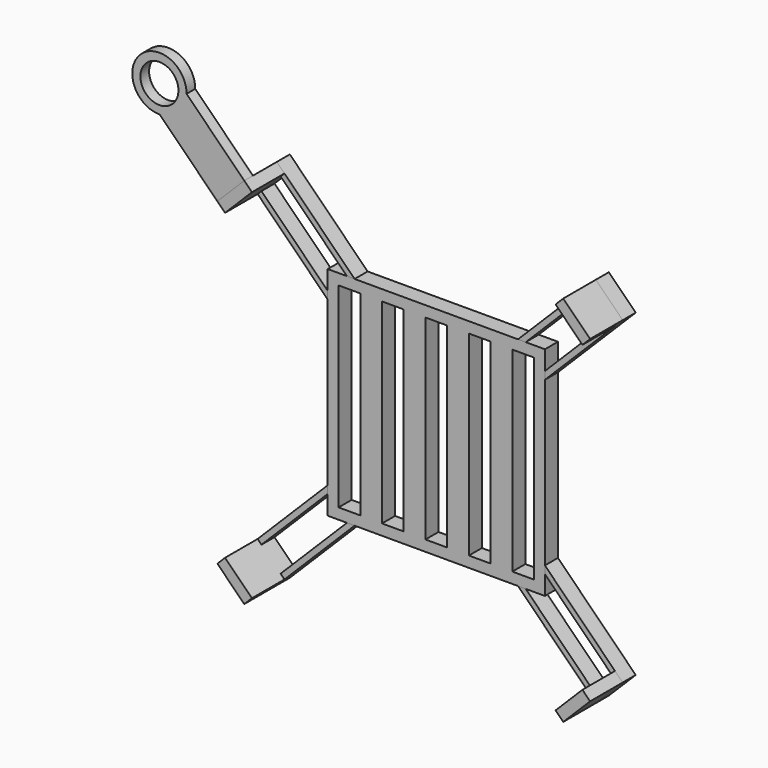
from build123d import *

# Parameters (mm, degrees)
F0_W      = 40
F0_H      = 40
F0_W_2    = 4
F0_H_2    = 36
F1_DEPTH  = 3
F3_DEPTH  = 3
F4_DEPTH  = 25
F5_DEPTH  = 25
F6_DEPTH  = 25
F7_DEPTH  = 25
F9_DEPTH  = 7.5
F10_R     = 3.5
F11_DEPTH = 2


# Not quite as in the source:
# - the program builds the solid bodies; features that only make, move or delete a surface that nothing else refers to are left out


with BuildPart() as f1:
    # F0 (on Front) → F1 (new body)
    with BuildSketch(Plane.XZ):
        Rectangle(F0_W, F0_H)
        with Locations((-16, 0)):
            Rectangle(F0_W_2, F0_H_2, mode=Mode.SUBTRACT)
        with Locations((-8, 0)):
            Rectangle(F0_W_2, F0_H_2, mode=Mode.SUBTRACT)
        Rectangle(F0_W_2, F0_H_2, mode=Mode.SUBTRACT)
        with Locations((8, 0)):
            Rectangle(F0_W_2, F0_H_2, mode=Mode.SUBTRACT)
        with Locations((16, 0)):
            Rectangle(F0_W_2, F0_H_2, mode=Mode.SUBTRACT)
    extrude(amount=F1_DEPTH)


with BuildPart() as f3:
    # F2 (on Front) → F3 (new body)
    with BuildSketch(Plane.XZ):
        Polygon((27.9616906966, 32.9114381649), (15.0502525317, 20), (16.4644660941, 20), (28.6687974778, 32.2043313837), align=None)
        Polygon((29.3759042589, 34.3256517272), (27.9616906966, 32.9114381649), (28.6687974778, 32.2043313837), (32.2043313837, 28.6687974778), (32.9114381649, 27.9616906966), (34.3256517272, 29.3759042589), align=None)
        Polygon((28.6687974778, 32.2043313837), (16.4644660941, 20), (20.0434662402, 20), (20.0125289488, 16.4769950429), (32.2043313837, 28.6687974778), align=None)
        Polygon((32.9114381649, 27.9616906966), (32.2043313837, 28.6687974778), (20.0125289488, 16.4769950429), (20, 15.0502525317), align=None)
    extrude(amount=F3_DEPTH)

    # F2 (on Front) → F4 (cut)
    with BuildSketch(Plane.XZ):
        Polygon((28.6687974778, 32.2043313837), (16.4644660941, 20), (20.0434662402, 20), (20.0125289488, 16.4769950429), (32.2043313837, 28.6687974778), align=None)
    extrude(amount=F4_DEPTH, mode=Mode.SUBTRACT)


with BuildPart() as f3b:
    # F2 (on Front) → F3, piece 2 (new body)
    with BuildSketch(Plane.XZ):
        Polygon((-16.4644660941, 20), (-28.6687974778, 32.2043313837), (-32.2043313837, 28.6687974778), (-20, 16.4644660941), (-20, 20), align=None)
        Polygon((-27.9616906966, 32.9114381649), (-28.6687974778, 32.2043313837), (-16.4644660941, 20), (-15.0502525317, 20), align=None)
        Polygon((-32.2043313837, 28.6687974778), (-28.6687974778, 32.2043313837), (-27.9616906966, 32.9114381649), (-29.3759042589, 34.3256517272), (-34.3256517272, 29.3759042589), (-32.9114381649, 27.9616906966), align=None)
        Polygon((-20, 16.4644660941), (-32.2043313837, 28.6687974778), (-32.9114381649, 27.9616906966), (-20, 15.0502525317), align=None)
    extrude(amount=F3_DEPTH)

    # F2 (on Front) → F5 (cut)
    with BuildSketch(Plane.XZ):
        Polygon((-16.4644660941, 20), (-28.6687974778, 32.2043313837), (-32.2043313837, 28.6687974778), (-20, 16.4644660941), (-20, 20), align=None)
    extrude(amount=F5_DEPTH, mode=Mode.SUBTRACT)


with BuildPart() as f3c:
    # F2 (on Front) → F3, piece 3 (new body)
    with BuildSketch(Plane.XZ):
        Polygon((-27.9616906966, -32.9114381649), (-28.6687974778, -32.2043313837), (-32.2043313837, -28.6687974778), (-32.9114381649, -27.9616906966), (-34.3256517272, -29.3759042589), (-29.3759042589, -34.3256517272), align=None)
        Polygon((-32.2043313837, -28.6687974778), (-28.6687974778, -32.2043313837), (-16.4644660941, -20), (-20, -20), (-20, -16.4644660941), align=None)
        Polygon((-16.4644660941, -20), (-28.6687974778, -32.2043313837), (-27.9616906966, -32.9114381649), (-15.0502525317, -20), align=None)
        Polygon((-32.9114381649, -27.9616906966), (-32.2043313837, -28.6687974778), (-20, -16.4644660941), (-20, -15.0502525317), align=None)
    extrude(amount=F3_DEPTH)

    # F2 (on Front) → F7 (cut)
    with BuildSketch(Plane.XZ):
        Polygon((-32.2043313837, -28.6687974778), (-28.6687974778, -32.2043313837), (-16.4644660941, -20), (-20, -20), (-20, -16.4644660941), align=None)
    extrude(amount=F7_DEPTH, mode=Mode.SUBTRACT)

    # F8 (on face) → F9 (join)
    with BuildSketch(Plane.XZ.offset(3)):
        Polygon((-34.3256517272, -29.3759042589), (-29.3759042589, -34.3256517272), (-27.9616906966, -32.9114381649), (-28.6687974778, -32.2043313837), (-32.2043313837, -28.6687974778), (-32.9114381649, -27.9616906966), align=None)
    extrude(amount=F9_DEPTH)


with BuildPart() as f3d:
    # F2 (on Front) → F3, piece 4 (new body)
    with BuildSketch(Plane.XZ):
        Polygon((16.4644660941, -20), (28.6687974778, -32.2043313837), (32.2043313837, -28.6687974778), (20, -16.4644660941), (20, -20), align=None)
        Polygon((27.9616906966, -32.9114381649), (28.6687974778, -32.2043313837), (16.4644660941, -20), (15.0502525317, -20), align=None)
        Polygon((32.2043313837, -28.6687974778), (28.6687974778, -32.2043313837), (27.9616906966, -32.9114381649), (29.3759042589, -34.3256517272), (34.3256517272, -29.3759042589), (32.9114381649, -27.9616906966), align=None)
        Polygon((20, -16.4644660941), (32.2043313837, -28.6687974778), (32.9114381649, -27.9616906966), (20, -15.0502525317), align=None)
    extrude(amount=F3_DEPTH)

    # F2 (on Front) → F6 (cut)
    with BuildSketch(Plane.XZ):
        Polygon((16.4644660941, -20), (28.6687974778, -32.2043313837), (32.2043313837, -28.6687974778), (20, -16.4644660941), (20, -20), align=None)
    extrude(amount=F6_DEPTH, mode=Mode.SUBTRACT)


with BuildPart() as f9:
    # F8 (on face) → F9, piece 2 (new body)
    with BuildSketch(Plane.XZ.offset(3)):
        Polygon((32.2043313837, -28.6687974778), (28.6687974778, -32.2043313837), (27.9616906966, -32.9114381649), (29.3759042589, -34.3256517272), (34.3256517272, -29.3759042589), (32.9114381649, -27.9616906966), align=None)
    extrude(amount=F9_DEPTH)


with BuildPart() as f9b:
    # F8 (on face) → F9, piece 3 (new body)
    with BuildSketch(Plane.XZ.offset(3)):
        Polygon((-27.9616906966, 32.9114381649), (-29.3759042589, 34.3256517272), (-34.3256517272, 29.3759042589), (-32.9114381649, 27.9616906966), (-32.2043313837, 28.6687974778), (-28.6687974778, 32.2043313837), align=None)
    extrude(amount=F9_DEPTH)


with BuildPart() as f9c:
    # F8 (on face) → F9, piece 4 (new body)
    with BuildSketch(Plane.XZ.offset(3)):
        Polygon((34.3256517272, 29.3759042589), (29.3759042589, 34.3256517272), (27.9616906966, 32.9114381649), (28.6687974778, 32.2043313837), (32.2043313837, 28.6687974778), (32.9114381649, 27.9616906966), align=None)
    extrude(amount=F9_DEPTH)


with BuildPart() as f11:
    # F10 (on face) → F11 (new body)
    with BuildSketch(Plane.XZ.offset(10.5)):
        with BuildLine():
            Line((-34.3256517272, 29.3759042589), (-29.3759042589, 34.3256517272))
            Line((-29.3759042589, 34.3256517272), (-40.0002500313, 44.9499974996))
            ThreePointArc((-40.0002500313, 44.9499974996), (-48.5355339059, 48.5355339059), (-44.9499974996, 40.0002500313))
            Line((-44.9499974996, 40.0002500313), (-34.3256517272, 29.3759042589))
        make_face()
        with Locations((-45, 45)):
            Circle(F10_R, mode=Mode.SUBTRACT)
    extrude(amount=-F11_DEPTH)


solid = Compound([f1.part, f3.part, f3b.part, f3c.part, f3d.part, f9.part, f9b.part, f9c.part, f11.part])
